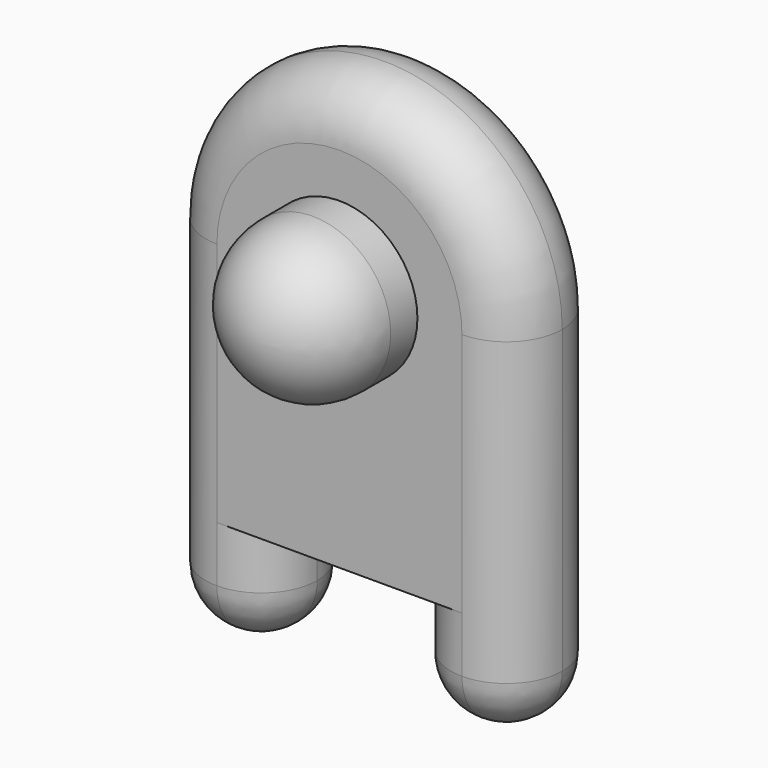
from build123d import *

# Parameters (mm, degrees)
F1_DEPTH     = 125
F2_R         = 175
F3_DEPTH     = 250
F4_R         = 124.99999
F5_T1_DEPTH  = 800
F5_T3_DEPTH  = 250
F5_T6_ANGLE  = 90
F5_T8_ANGLE  = 90
F5_T10_ANGLE = 90
F5_T12_ANGLE = 90
F5_T14_ANGLE = 90
F5_T16_ANGLE = 90
F5_T18_ANGLE = 90
F5_T20_ANGLE = 90
F5_T22_ANGLE = 180
F5_T24_ANGLE = 180
F6_R         = 175


# Not quite as in the source:
# - a fillet or chamfer that OpenCascade refuses, or shapes differently, is made with other operations: its cross-section is extruded or revolved along the edge and cut away or added
# - a fillet or chamfer is up to 0.001 mm smaller than in the source, because OpenCascade refuses the exact size


with BuildPart() as f1:
    # F0 (on Front) → F1 (new body, symmetric)
    with BuildSketch(Plane.XZ):
        with BuildLine():
            Line((400, -800), (400, 0))
            ThreePointArc((400, 0), (0, 400), (-400, 0))
            Line((-400, 0), (-400, -800))
            Line((-400, -800), (-150, -800))
            Line((-150, -800), (-150, -550))
            Line((-150, -550), (150, -550))
            Line((150, -550), (150, -800))
            Line((150, -800), (400, -800))
        make_face()
    extrude(amount=F1_DEPTH, both=True)

    # F2 (on face) → F3 (join, symmetric)
    with BuildSketch(Plane.XZ.offset(125)):
        Circle(F2_R)
    extrude(amount=F3_DEPTH, both=True)

    # F4 (radius 125 in the source; OpenCascade refuses exactly that, so slightly less here)
    f4_edges = [f1.edges().sort_by_distance(p)[0] for p in [
        (-400, 0, -800),
        (-275, 125, -800),
        (-150, 0, -800),
        (-275, -125, -800),
        (150, 0, -800),
        (275, 125, -800),
        (400, 0, -800),
        (275, -125, -800),
    ]]
    fillet(f4_edges, radius=F4_R)

    # F5: fillet of radius 125 on 8 edges, made by hand

    # F5_s2 → F5_t1 (cut)
    with BuildSketch(Plane.XY.offset(-800)):
        with BuildLine():
            ThreePointArc((275, -125), (363.3883476483, -88.3883476483), (400, 0))
            Line((400, 0), (400, -125))
            Line((400, -125), (275, -125))
        make_face()
        with BuildLine():
            ThreePointArc((275, 125), (363.3883476483, 88.3883476483), (400, 0))
            Line((400, 0), (400, 125))
            Line((400, 125), (275, 125))
        make_face()
        with BuildLine():
            ThreePointArc((-400, 0), (-363.3883476483, -88.3883476483), (-275, -125))
            Line((-275, -125), (-400, -125))
            Line((-400, -125), (-400, 0))
        make_face()
        with BuildLine():
            ThreePointArc((-400, 0), (-363.3883476483, 88.3883476483), (-275, 125))
            Line((-275, 125), (-400, 125))
            Line((-400, 125), (-400, 0))
        make_face()
    extrude(amount=F5_T1_DEPTH, mode=Mode.SUBTRACT)

    # F5_s4 → F5_t3 (cut)
    with BuildSketch(Plane.XY.offset(-800)):
        with BuildLine():
            ThreePointArc((-275, 125), (-186.6116523517, 88.3883476483), (-150, 0))
            Line((-150, 0), (-150, 125))
            Line((-150, 125), (-275, 125))
        make_face()
        with BuildLine():
            ThreePointArc((-275, -125), (-186.6116523517, -88.3883476483), (-150, 0))
            Line((-150, 0), (-150, -125))
            Line((-150, -125), (-275, -125))
        make_face()
        with BuildLine():
            ThreePointArc((275, -125), (186.6116523517, -88.3883476483), (150, 0))
            Line((150, 0), (150, -125))
            Line((150, -125), (275, -125))
        make_face()
        with BuildLine():
            ThreePointArc((275, 125), (186.6116523517, 88.3883476483), (150, 0))
            Line((150, 0), (150, 125))
            Line((150, 125), (275, 125))
        make_face()
    extrude(amount=F5_T3_DEPTH, mode=Mode.SUBTRACT)

    # F5_s5 → F5_t6 (revolve, cut)
    with BuildSketch(Plane.XZ):
        with BuildLine():
            ThreePointArc((274.99999, -800), (186.6116494227, -763.3883505773), (150, -675.00001))
            Line((150, -675.00001), (150, -800))
            Line((150, -800), (274.99999, -800))
        make_face()
    revolve(axis=Axis((275, 0, -800), (0, 0, -1)), revolution_arc=F5_T6_ANGLE, mode=Mode.SUBTRACT)

    # F5_s7 → F5_t8 (revolve, cut)
    with BuildSketch(Plane.YZ.offset(275)):
        with BuildLine():
            ThreePointArc((-1e-05, -800), (-88.3883505773, -763.3883505773), (-125, -675.00001))
            Line((-125, -675.00001), (-125, -800))
            Line((-125, -800), (-1e-05, -800))
        make_face()
    revolve(axis=Axis((275, 0, -800), (0, 0, -1)), revolution_arc=F5_T8_ANGLE, mode=Mode.SUBTRACT)

    # F5_s9 → F5_t10 (revolve, cut)
    with BuildSketch(Plane.XZ):
        with BuildLine():
            ThreePointArc((-274.99999, -800), (-186.6116494227, -763.3883505773), (-150, -675.00001))
            Line((-150, -675.00001), (-150, -800))
            Line((-150, -800), (-274.99999, -800))
        make_face()
    revolve(axis=Axis((-275, 0, -800), (0, 0, -1)), revolution_arc=F5_T10_ANGLE, mode=Mode.SUBTRACT)

    # F5_s11 → F5_t12 (revolve, cut)
    with BuildSketch(Plane.YZ.offset(-275)):
        with BuildLine():
            ThreePointArc((1e-05, -800), (88.3883505773, -763.3883505773), (125, -675.00001))
            Line((125, -675.00001), (125, -800))
            Line((125, -800), (1e-05, -800))
        make_face()
    revolve(axis=Axis((-275, 0, -800), (0, 0, -1)), revolution_arc=F5_T12_ANGLE, mode=Mode.SUBTRACT)

    # F5_s13 → F5_t14 (revolve, cut)
    with BuildSketch(Plane.XZ):
        with BuildLine():
            ThreePointArc((-275.00001, -800), (-363.3883505773, -763.3883505773), (-400, -675.00001))
            Line((-400, -675.00001), (-400, -800))
            Line((-400, -800), (-275.00001, -800))
        make_face()
    revolve(axis=Axis((-275, 0, -800), (0, 0, -1)), revolution_arc=F5_T14_ANGLE, mode=Mode.SUBTRACT)

    # F5_s15 → F5_t16 (revolve, cut)
    with BuildSketch(Plane.YZ.offset(-275)):
        with BuildLine():
            ThreePointArc((-1e-05, -800), (-88.3883505773, -763.3883505773), (-125, -675.00001))
            Line((-125, -675.00001), (-125, -800))
            Line((-125, -800), (-1e-05, -800))
        make_face()
    revolve(axis=Axis((-275, 0, -800), (0, 0, -1)), revolution_arc=F5_T16_ANGLE, mode=Mode.SUBTRACT)

    # F5_s17 → F5_t18 (revolve, cut)
    with BuildSketch(Plane.YZ.offset(275)):
        with BuildLine():
            ThreePointArc((1e-05, -800), (88.3883505773, -763.3883505773), (125, -675.00001))
            Line((125, -675.00001), (125, -800))
            Line((125, -800), (1e-05, -800))
        make_face()
    revolve(axis=Axis((275, 0, -800), (0, 0, -1)), revolution_arc=F5_T18_ANGLE, mode=Mode.SUBTRACT)

    # F5_s19 → F5_t20 (revolve, cut)
    with BuildSketch(Plane.XZ):
        with BuildLine():
            ThreePointArc((275.00001, -800), (363.3883505773, -763.3883505773), (400, -675.00001))
            Line((400, -675.00001), (400, -800))
            Line((400, -800), (275.00001, -800))
        make_face()
    revolve(axis=Axis((275, 0, -800), (0, 0, -1)), revolution_arc=F5_T20_ANGLE, mode=Mode.SUBTRACT)

    # F5_s21 → F5_t22 (revolve, cut)
    with BuildSketch(Plane.XY):
        with BuildLine():
            ThreePointArc((275, 125), (363.3883476483, 88.3883476483), (400, 0))
            Line((400, 0), (400, 125))
            Line((400, 125), (275, 125))
        make_face()
    revolve(axis=Axis((0, 125, 0), (0, -1, 0)), revolution_arc=F5_T22_ANGLE, mode=Mode.SUBTRACT)

    # F5_s23 → F5_t24 (revolve, cut)
    with BuildSketch(Plane.XY):
        with BuildLine():
            ThreePointArc((400, 0), (363.3883476483, -88.3883476483), (275, -125))
            Line((275, -125), (400, -125))
            Line((400, -125), (400, 0))
        make_face()
    revolve(axis=Axis((0, -125, 0), (0, -1, 0)), revolution_arc=F5_T24_ANGLE, mode=Mode.SUBTRACT)

    # F6
    f6_edges = [f1.edges().sort_by_distance(p)[0] for p in [
        (-175, -375, 0),
    ]]
    fillet(f6_edges, radius=F6_R)


solid = f1.part
